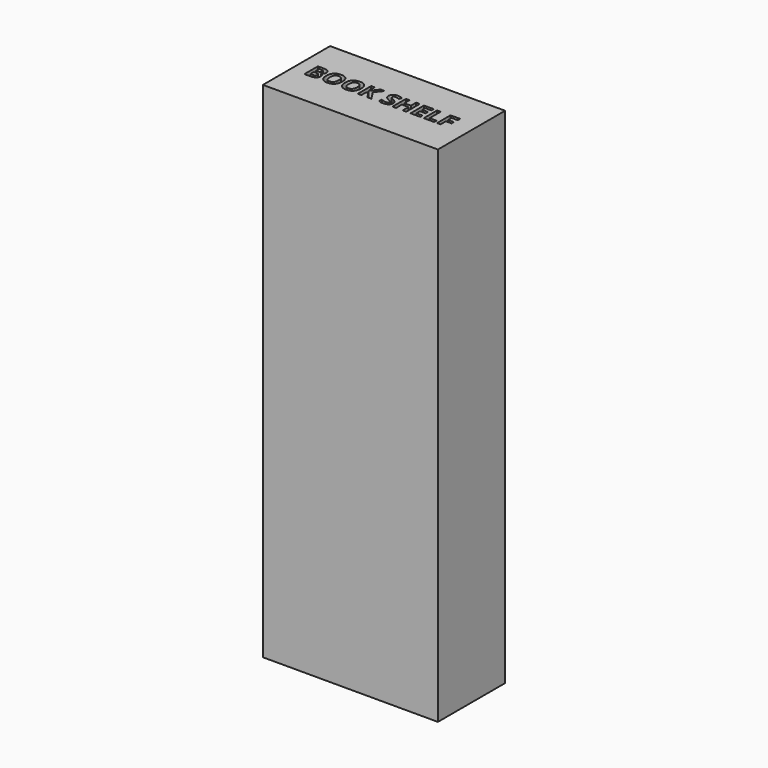
from build123d import *

# Parameters (mm, degrees)
F0_W         = 635
F0_H         = 304.8
F1_DEPTH     = 1828.8
F2_TEXT_SIZE = 85.4955779182
F3_DEPTH     = 25.4


# Not quite as in the source:
# - Text() gives the source's letters only with a copy of the font that has no kerning and outlines rounded to 1/6400 em; it was checked with that copy


with BuildPart() as f1:
    # F0 (on Top) → F1 (new body)
    with BuildSketch(Plane.XY):
        with Locations((317.5, 152.4)):
            Rectangle(F0_W, F0_H)
    extrude(amount=F1_DEPTH)

    # F2 (on face) → F3 (cut)
    with BuildSketch(Plane.XY.offset(1828.8)):
        with Locations((42.8734514862, 125.1443326473)):
            Text('BOOK SHELF', F2_TEXT_SIZE, font='Open Sans', font_style=FontStyle.BOLD, text_align=(TextAlign.LEFT, TextAlign.BOTTOM))
    extrude(amount=-F3_DEPTH, mode=Mode.SUBTRACT)


solid = f1.part
